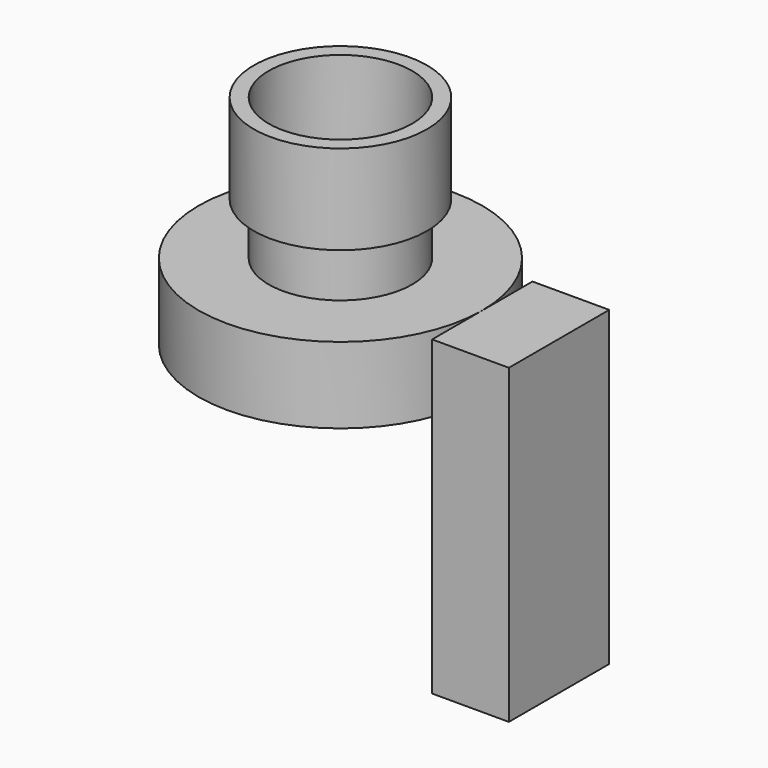
from build123d import *

# Parameters (mm, degrees)
F0_R     = 2.4
F1_DEPTH = 1.74
F2_R     = 2.9
F2_R_2   = 2.4
F3_DEPTH = 3
F4_R     = 4.75
F4_R_2   = 2.4
F5_DEPTH = 2.55
F8_DEPTH = 2.57


with BuildPart() as f1:
    # F0 (on Top) → F1 (new body)
    with BuildSketch(Plane.XY):
        Circle(F0_R)
    extrude(amount=F1_DEPTH)


with BuildPart() as f3:
    # F2 (on face) → F3 (new body)
    with BuildSketch(Plane.XY.offset(1.74)):
        Circle(F2_R)
        Circle(F2_R_2, mode=Mode.SUBTRACT)
    extrude(amount=F3_DEPTH)


with BuildPart() as f5:
    # F4 (on face) → F5 (new body)
    with BuildSketch(Plane(origin=(0, 0, 0), x_dir=(1, 0, 0), z_dir=(0, 0, -1))):
        Circle(F4_R)
        Circle(F4_R_2, mode=Mode.SUBTRACT)
        Circle(F4_R_2)
    extrude(amount=F5_DEPTH)


with BuildPart() as f8:
    # F7 (on offset) → F8 (new body)
    with BuildSketch(Plane.YZ.offset(4.75)):
        Polygon((2.1, 0), (0, 0), (-2.1, 0), (-2.1, -10.44), (2.1, -10.44), align=None)
    extrude(amount=F8_DEPTH)


solid = Compound([f1.part, f3.part, f5.part, f8.part])
